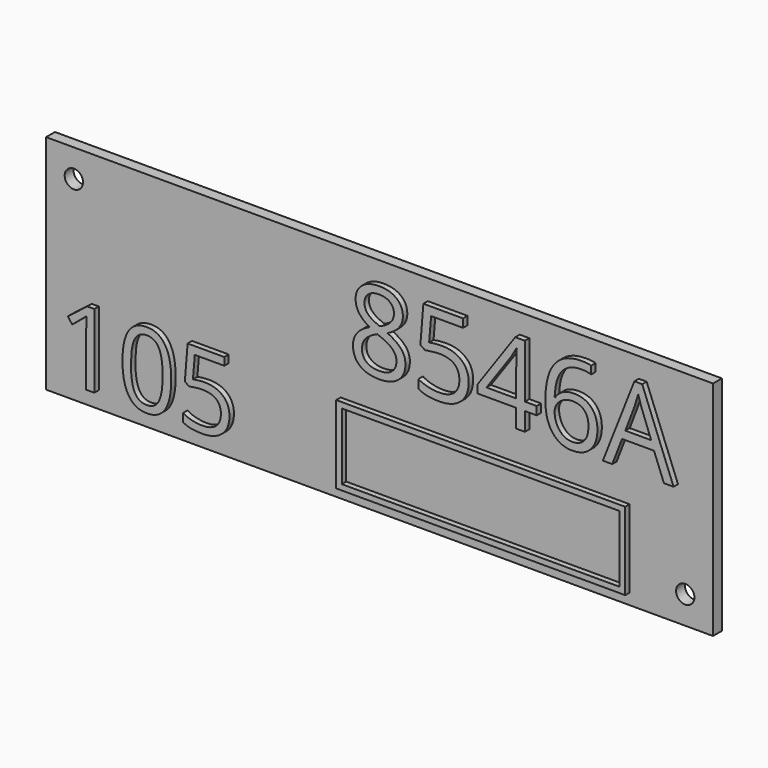
from build123d import *

# Parameters (mm, degrees)
F0_W         = 120
F0_H         = 40
F1_DEPTH     = 2
F3_D         = 3.3
F4_TEXT_SIZE = 20.1036594943
F5_DEPTH     = 1
F6_TEXT_SIZE = 18.5776487663
F7_DEPTH     = 1
F8_W         = 52
F8_H         = 14
F8_W_2       = 49.99999962
F8_H_2       = 11.99999962
F9_DEPTH     = 1


# Not quite as in the source:
# - Text() gives the source's letters only with a copy of the font that has no kerning and outlines rounded to 1/6400 em; it was checked with that copy


with BuildPart() as f1:
    # F0 (on Front) → F1 (new body)
    with BuildSketch(Plane.XZ):
        Rectangle(F0_W, F0_H)
    extrude(amount=F1_DEPTH)

    # F3 (through all)
    with Locations(Plane.XZ.offset(2)):
        with Locations((-55, 15), (55, -15)):
            Hole(F3_D / 2)

    # F4 (on face) → F5 (join)
    with BuildSketch(Plane.XZ.offset(2)):
        with Locations((-5, 2)):
            Text('8546A', F4_TEXT_SIZE, font='Open Sans', text_align=(TextAlign.LEFT, TextAlign.BOTTOM))
    extrude(amount=F5_DEPTH)

    # F6 (on face) → F7 (join)
    with BuildSketch(Plane.XZ.offset(2)):
        with Locations((-57, -17)):
            Text('105', F6_TEXT_SIZE, font='Open Sans', text_align=(TextAlign.LEFT, TextAlign.BOTTOM))
    extrude(amount=F7_DEPTH)

    # F8 (on face) → F9 (join)
    with BuildSketch(Plane.XZ.offset(2)):
        with Locations((19, -11)):
            Rectangle(F8_W, F8_H)
        with Locations((19, -11)):
            Rectangle(F8_W_2, F8_H_2, mode=Mode.SUBTRACT)
    extrude(amount=F9_DEPTH)


solid = f1.part
